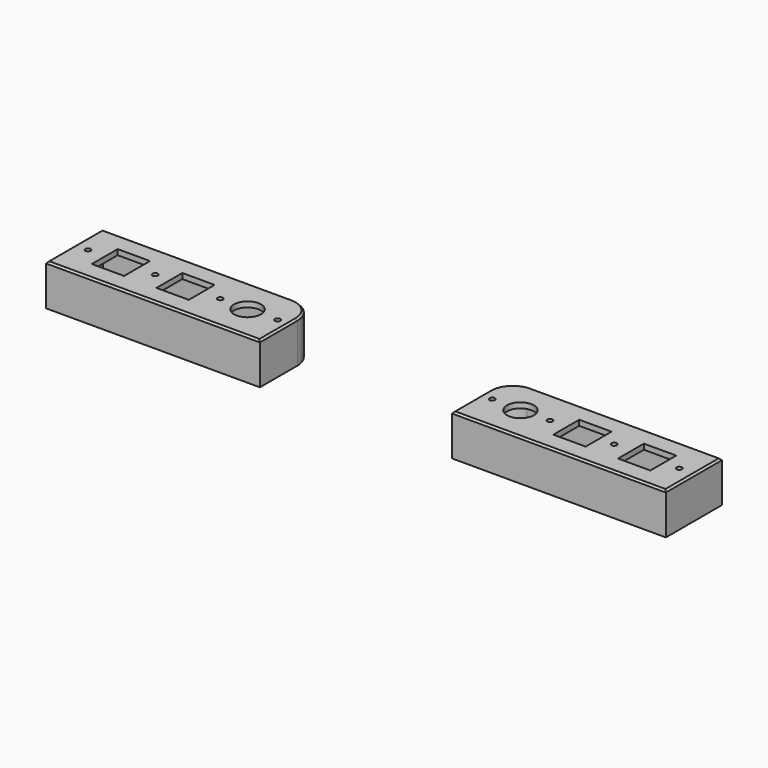
from build123d import *

# Parameters (mm, degrees)
F1_DEPTH      = 5
F1_DEPTH_BACK = 15
F2_T          = 3
F2_2_T        = 3
F4_W          = 18
F4_H          = 18
F4_R          = 7.5
F5_DEPTH      = 50
F8_D          = 3
F8_DEPTH      = 40
F8_TIP        = 0.9012909285
F8_2_D        = 3
F8_2_DEPTH    = 40
F8_2_TIP      = 0.9012909285
F9_SIZE       = 1
F9_2_SIZE     = 1


with BuildPart() as f1:
    # F0 (on Top) → F1 (new body, two sides)
    with BuildSketch(Plane.XY) as f1_sk:
        with BuildLine():
            Line((169.1123094261, 78.8974409995), (66.1123094261, 78.8974409995))
            ThreePointArc((66.1123094261, 78.8974409995), (59.0412416142, 75.9685088113), (56.1123094261, 68.8974409995))
            Line((56.1123094261, 68.8974409995), (56.1123094261, 45.8974409995))
            Line((56.1123094261, 45.8974409995), (169.1123094261, 45.8974409995))
            Line((169.1123094261, 45.8974409995), (169.1123094261, 78.8974409995))
        make_face()
    extrude(amount=F1_DEPTH)
    extrude(f1_sk.sketch, amount=-F1_DEPTH_BACK)

    # F2
    f2_openings = [f1.faces().sort_by_distance(p)[0] for p in [
        (112.926417, 62.314864, -15),
    ]]
    offset(amount=F2_T, openings=f2_openings, kind=Kind.INTERSECTION)


with BuildPart() as f1b:
    # F0 (on Top) → F1, piece 2 (new body, two sides)
    with BuildSketch(Plane.XY) as f1_2_sk:
        with BuildLine():
            Line((-66.9198182523, 78.9953285099), (-169.9198182523, 78.9953285099))
            Line((-169.9198182523, 78.9953285099), (-169.9198182523, 45.9953285099))
            Line((-169.9198182523, 45.9953285099), (-56.9198182523, 45.9953285099))
            Line((-56.9198182523, 45.9953285099), (-56.9198182523, 68.9953285099))
            ThreePointArc((-56.9198182523, 68.9953285099), (-59.8487504405, 76.0663963218), (-66.9198182523, 78.9953285099))
        make_face()
    extrude(amount=F1_DEPTH)
    extrude(f1_2_sk.sketch, amount=-F1_DEPTH_BACK)

    # F2#2
    f2_2_openings = [f1b.faces().sort_by_distance(p)[0] for p in [
        (-113.733926, 62.412751, -15),
    ]]
    offset(amount=F2_2_T, openings=f2_2_openings, kind=Kind.INTERSECTION)


with BuildPart() as f5_tool:
    # F4 (on offset) → F5 (new body)
    with BuildSketch(Plane.XY.offset(33)):
        with Locations((-146.8929139701, 62.4953285099)):
            Rectangle(F4_W, F4_H)
        with Locations((-110.8929139701, 62.4953285099)):
            Rectangle(F4_W, F4_H)
        with Locations((-76.3929139701, 62.4953285099)):
            Circle(F4_R)
        with Locations((75.5820007977, 62.3974409995)):
            Circle(F4_R)
        with Locations((110.0820007977, 62.3974409995)):
            Rectangle(F4_W, F4_H)
        with Locations((146.0820007977, 62.3974409995)):
            Rectangle(F4_W, F4_H)
    extrude(amount=-F5_DEPTH)


with BuildPart() as f1_1:
    add(f1.part)

    # F5: cut by f5_tool
    add(f5_tool.part, mode=Mode.SUBTRACT)

    # F8
    with Locations(Plane.XY.offset(8)):
        with Locations((-128.1331330538, 62.8871805966), (163.6322605932, 62.8871805966), (127.36319817, 62.8871805966), (-165.489256382, 62.8871805966), (91.6408523917, 62.8871805966), (59.4655014575, 62.8871805966), (-91.8687133804, 62.8871805966), (-59.9663094311, 62.8871805966)):
            Hole(F8_D / 2, depth=F8_DEPTH)
            with Locations((0, 0, -(F8_DEPTH + F8_TIP / 2))):  # 118° drill point
                Cone(0, F8_D / 2, F8_TIP, mode=Mode.SUBTRACT)

    # F9
    f9_edges = [f1_1.edges().sort_by_distance(p)[0] for p in [
        (112.612309, 42.897441, 8),
        (172.112309, 62.397441, 8),
        (119.112309, 81.897441, 8),
        (56.919921, 78.089829, 8),
        (53.112309, 55.897441, 8),
    ]]
    chamfer(f9_edges, length=F9_SIZE)


with BuildPart() as f1b_1:
    add(f1b.part)

    # F5: cut by f5_tool
    add(f5_tool.part, mode=Mode.SUBTRACT)

    # F8#2
    with Locations(Plane.XY.offset(8)):
        with Locations((-128.1331330538, 62.8871805966), (163.6322605932, 62.8871805966), (127.36319817, 62.8871805966), (-165.489256382, 62.8871805966), (91.6408523917, 62.8871805966), (59.4655014575, 62.8871805966), (-91.8687133804, 62.8871805966), (-59.9663094311, 62.8871805966)):
            Hole(F8_2_D / 2, depth=F8_2_DEPTH)
            with Locations((0, 0, -(F8_2_DEPTH + F8_2_TIP / 2))):  # 118° drill point
                Cone(0, F8_2_D / 2, F8_2_TIP, mode=Mode.SUBTRACT)

    # F9#2
    f9_2_edges = [f1b_1.edges().sort_by_distance(p)[0] for p in [
        (-53.919818, 55.995329, 8),
        (-57.72743, 78.187717, 8),
        (-119.919818, 81.995329, 8),
        (-172.919818, 62.495329, 8),
        (-113.419818, 42.995329, 8),
    ]]
    chamfer(f9_2_edges, length=F9_2_SIZE)


solid = Compound([f1_1.part, f1b_1.part])
